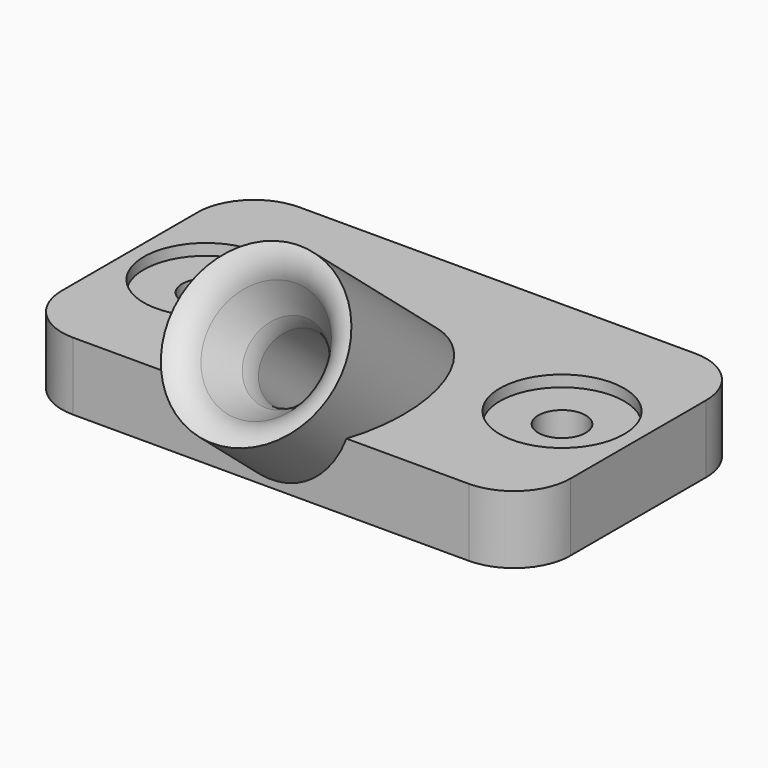
from build123d import *

# Parameters (mm, degrees)
F0_W           = 45
F0_H           = 25
F1_DEPTH       = 6
F2_R           = 5
F4_R           = 5.5
F5_DEPTH       = 25
F6_R           = 2.1
F7_DEPTH       = 25
F9_R           = 7.5
F10_DEPTH      = 5
F10_DEPTH_BACK = 25
F11_W          = 49.2877000943
F11_H          = 30.2235903218
F12_DEPTH      = 25
F13_W          = 37.6632460393
F13_H          = 10.6945014559
F14_DEPTH      = 25
F15_R          = 3
F16_DEPTH      = 25
F16_DEPTH_BACK = 25
F18_R          = 3


# Not quite as in the source:
# - a fillet or chamfer that OpenCascade refuses, or shapes differently, is made with other operations: its cross-section is extruded or revolved along the edge and cut away or added


with BuildPart() as f1:
    # F0 (on Top) → F1 (new body)
    with BuildSketch(Plane.XY):
        with Locations((22.5, 12.5)):
            Rectangle(F0_W, F0_H)
    extrude(amount=F1_DEPTH)

    # F2
    f2_edges = [f1.edges().sort_by_distance(p)[0] for p in [
        (45, 25, 3),
        (45, 0, 3),
        (0, 25, 3),
        (0, 0, 3),
    ]]
    fillet(f2_edges, radius=F2_R)

    # F4 (on offset) → F5 (cut)
    with BuildSketch(Plane.XY.offset(5)):
        with Locations((6.75, 12.5)):
            Circle(F4_R)
        with Locations((38.25, 12.5)):
            Circle(F4_R)
    extrude(amount=F5_DEPTH, mode=Mode.SUBTRACT)

    # F6 (on Top) → F7 (cut)
    with BuildSketch(Plane.XY):
        with Locations((6.75, 12.5)):
            Circle(F6_R)
        with Locations((38.25, 12.5)):
            Circle(F6_R)
    extrude(amount=F7_DEPTH, mode=Mode.SUBTRACT)

    # F9 (on face) → F10 (join, two sides)
    with BuildSketch(Plane(origin=(0, -2.954423259, 2.479055467), x_dir=(1, 0, 0), z_dir=(0, -0.7660444431, 0.6427876097))) as f10_sk:
        with Locations((22.5, 8)):
            Circle(F9_R)
    extrude(amount=F10_DEPTH)
    extrude(f10_sk.sketch, amount=-F10_DEPTH_BACK)

    # F11 (on Top) → F12 (cut)
    with BuildSketch(Plane.XY):
        with Locations((22.6797270589, 13.7661970221)):
            Rectangle(F11_W, F11_H)
    extrude(amount=-F12_DEPTH, mode=Mode.SUBTRACT)

    # F13 (on face) → F14 (cut)
    with BuildSketch(Plane(origin=(0, 25, 0), x_dir=(-1, 0, 0), z_dir=(0, 1, 0))):
        with Locations((-22.6992729586, 2.3689556401)):
            Rectangle(F13_W, F13_H)
    extrude(amount=F14_DEPTH, mode=Mode.SUBTRACT)

    # F15 (on face) → F16 (cut, two sides)
    with BuildSketch(Plane(origin=(0, -2.954423259, 2.479055467), x_dir=(1, 0, 0), z_dir=(0, -0.7660444431, 0.6427876097))) as f16_sk:
        with Locations((22.5, 8)):
            Circle(F15_R)
    extrude(amount=F16_DEPTH, mode=Mode.SUBTRACT)
    extrude(f16_sk.sketch, amount=-F16_DEPTH_BACK, mode=Mode.SUBTRACT)

    # F17: chamfer of 3 x 5 on 1 edges, made by hand

    # F17_s1 → F17_t2 (revolve, cut)
    with BuildSketch(Plane(origin=(0, 5.1423008775, 6.128355545), x_dir=(1, 0, 0), z_dir=(0, 0.6427876097, 0.7660444431))):
        Polygon((28.5, -8.8567256581), (25.5, -3.8567256581), (25.5, -8.8567256581), align=None)
    revolve(axis=Axis((22.5, -1.6423445971, 11.8213490604), (0, 0.7660444431, -0.6427876097)), mode=Mode.SUBTRACT)

    # F18
    f18_edges = [f1.edges().sort_by_distance(p)[0] for p in [
        (19.5, 2.187878, 8.607411),
    ]]
    fillet(f18_edges, radius=F18_R)

    # F19: fillet of radius 3 on 1 edges, made by hand

    # F19_s1 → F19_t2 (revolve, cut)
    with BuildSketch(Plane(origin=(0, 5.1423008775, 6.128355545), x_dir=(1, 0, 0), z_dir=(0, 0.6427876097, 0.7660444431))):
        with BuildLine():
            ThreePointArc((27.6302051352, -7.4070675501), (28.6371938466, -8.4227287465), (30, -8.8567256581))
            Line((30, -8.8567256581), (28.5, -8.8567256581))
            Line((28.5, -8.8567256581), (27.6302051352, -7.4070675501))
        make_face()
    revolve(axis=Axis((22.5, -1.6423445971, 11.8213490604), (0, 0.7660444431, -0.6427876097)), mode=Mode.SUBTRACT)


solid = f1.part
